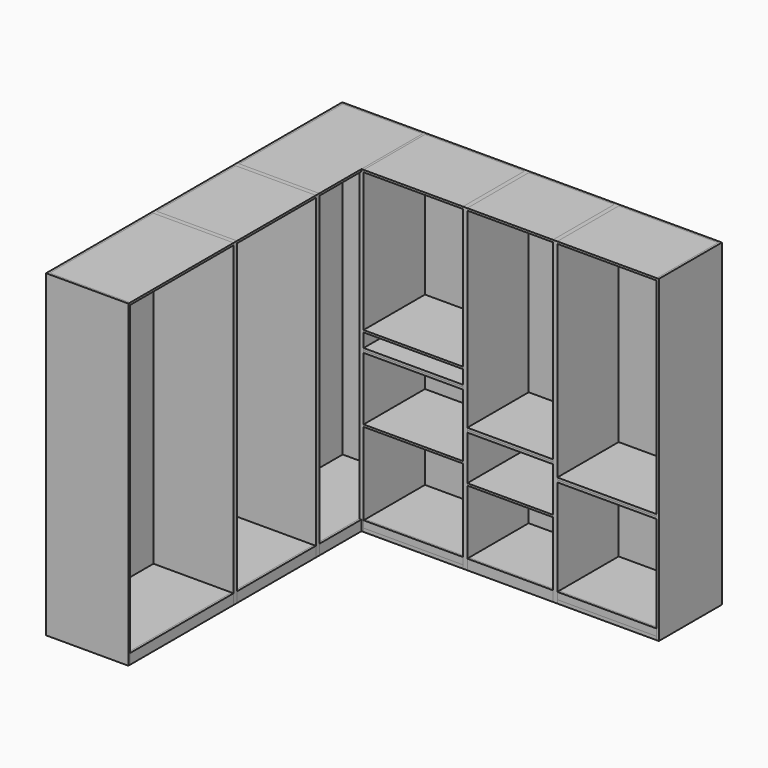
from build123d import *

# Parameters (mm, degrees)
F0_W      = 577.85
F0_H      = 730.25
F1_DEPTH  = 15.875
F0_W_2    = 736.6
F0_H_2    = 552.45
F0_W_3    = 635
F0_W_4    = 15.875
F0_H_3    = 958.85
F0_H_4    = 568.325
F0_H_5    = 15.875
F2_DEPTH  = 2362.2
F0_H_6    = 390.525
F3_DEPTH  = 76.2
F4_START  = 60.325
F4_DEPTH  = 15.875
F5_START  = 2346.325
F5_DEPTH  = 15.875
F6_DEPTH  = 25.4
F7_START  = 685.8
F7_DEPTH  = 15.875
F8_START  = 1168.4
F8_DEPTH  = 15.875
F9_START  = 1184.275
F9_DEPTH  = 15.875
F10_START = 1301.75
F10_DEPTH = 15.875
F11_START = 552.45
F11_DEPTH = 15.875
F12_START = 898.525
F12_DEPTH = 15.875
F13_START = 914.4
F13_DEPTH = 15.875
F14_DEPTH = 25.4
F15_START = 790.575
F15_DEPTH = 15.875
F16_START = 806.45
F16_DEPTH = 15.875
F17_R     = 12.7
F18_DEPTH = 768.35


# Not quite as in the source:
# - the program builds the solid bodies; features that only make, move or delete a surface that nothing else refers to are left out


with BuildPart() as f1:
    # F0 (on Top) → F1 (new body)
    with BuildSketch(Plane.XY):
        with Locations((-688.975, -1079.5)):
            Rectangle(F0_W, F0_H)
    extrude(amount=F1_DEPTH)


with BuildPart() as f1b:
    # F0 (on Top) → F1, piece 2 (new body)
    with BuildSketch(Plane.XY):
        Polygon((-400.05, -1866.9), (-400.05, -1476.375), (-977.9, -1476.375), (-977.9, -2435.225), (-400.05, -2435.225), align=None)
    extrude(amount=F1_DEPTH)


with BuildPart() as f1c:
    # F0 (on Top) → F1, piece 3 (new body)
    with BuildSketch(Plane.XY):
        Polygon((-400.05, -292.1), (-400.05, 276.225), (-977.9, 276.225), (-977.9, -682.625), (-400.05, -682.625), align=None)
    extrude(amount=F1_DEPTH)


with BuildPart() as f1d:
    # F0 (on Top) → F1, piece 4 (new body)
    with BuildSketch(Plane.XY):
        Rectangle(F0_W_2, F0_H_2)
    extrude(amount=F1_DEPTH)


with BuildPart() as f1e:
    # F0 (on Top) → F1, piece 5 (new body)
    with BuildSketch(Plane.XY):
        with Locations((717.55, 0)):
            Rectangle(F0_W_3, F0_H_2)
    extrude(amount=F1_DEPTH)


with BuildPart() as f1f:
    # F0 (on Top) → F1, piece 6 (new body)
    with BuildSketch(Plane.XY):
        with Locations((1435.1, 0)):
            Rectangle(F0_W_2, F0_H_2)
    extrude(amount=F1_DEPTH)


with BuildPart() as f2:
    # F0 (on Top) → F2 (new body)
    with BuildSketch(Plane.XY):
        Polygon((-977.9, -2435.225), (-993.775, -2435.225), (-993.775, -2451.1), (-384.175, -2451.1), (-384.175, -2435.225), (-400.05, -2435.225), align=None)
        with Locations((-985.8375, -1955.8)):
            Rectangle(F0_W_4, F0_H_3)
        Polygon((-384.175, -1476.375), (-384.175, -1460.5), (-993.775, -1460.5), (-993.775, -1476.375), (-977.9, -1476.375), (-400.05, -1476.375), align=None)
        Polygon((-384.175, -1460.5), (-384.175, -1444.625), (-400.05, -1444.625), (-977.9, -1444.625), (-993.775, -1444.625), (-993.775, -1460.5), align=None)
        with Locations((-985.8375, -1079.5)):
            Rectangle(F0_W_4, F0_H)
        Polygon((-384.175, -714.375), (-384.175, -698.5), (-993.775, -698.5), (-993.775, -714.375), (-977.9, -714.375), (-400.05, -714.375), align=None)
        Polygon((-384.175, -698.5), (-384.175, -682.625), (-400.05, -682.625), (-977.9, -682.625), (-993.775, -682.625), (-993.775, -698.5), align=None)
        with Locations((-392.1125, -7.9375)):
            Rectangle(F0_W_4, F0_H_4)
        Polygon((-368.3, 276.225), (-368.3, 292.1), (-384.175, 292.1), (-384.175, 276.225), (-384.175, -292.1), (-368.3, -292.1), (-368.3, -276.225), align=None)
        with Locations((-985.8375, -203.2)):
            Rectangle(F0_W_4, F0_H_3)
        Polygon((-384.175, 276.225), (-384.175, 292.1), (-993.775, 292.1), (-993.775, 276.225), (-977.9, 276.225), (-400.05, 276.225), align=None)
        with Locations((0, 284.1625)):
            Rectangle(F0_W_2, F0_H_5)
        Polygon((384.175, -292.1), (384.175, 292.1), (368.3, 292.1), (368.3, 276.225), (368.3, -276.225), (368.3, -292.1), align=None)
        Polygon((400.05, 292.1), (384.175, 292.1), (384.175, -292.1), (400.05, -292.1), (400.05, -276.225), (400.05, 276.225), align=None)
        with Locations((717.55, 284.1625)):
            Rectangle(F0_W_3, F0_H_5)
        Polygon((1050.925, 292.1), (1035.05, 292.1), (1035.05, 276.225), (1035.05, -276.225), (1035.05, -292.1), (1050.925, -292.1), align=None)
        Polygon((1066.8, 292.1), (1050.925, 292.1), (1050.925, -292.1), (1066.8, -292.1), (1066.8, -276.225), (1066.8, 276.225), align=None)
        with Locations((1435.1, 284.1625)):
            Rectangle(F0_W_2, F0_H_5)
        Polygon((1819.275, 292.1), (1803.4, 292.1), (1803.4, 276.225), (1803.4, -276.225), (1803.4, -292.1), (1819.275, -292.1), align=None)
    extrude(amount=F2_DEPTH)

    # F0 (on Top) → F15 (join)
    with BuildSketch(Plane.XY.offset(F15_START)):
        with Locations((1435.1, 0)):
            Rectangle(F0_W_2, F0_H_2)
        with Locations((1435.1, -284.1625)):
            Rectangle(F0_W_2, F0_H_5)
    extrude(amount=F15_DEPTH)

    # F17 (on face) → F18 (join)
    with BuildSketch(Plane.YZ.offset(1819.275)):
        with Locations((0, 2199.675321579)):
            Circle(F17_R)
    extrude(amount=-F18_DEPTH)


with BuildPart() as f3:
    # F0 (on Top) → F3 (new body)
    with BuildSketch(Plane.XY):
        with Locations((-392.1125, -2151.0625)):
            Rectangle(F0_W_4, F0_H_4)
        with Locations((-392.1125, -1671.6375)):
            Rectangle(F0_W_4, F0_H_6)
    extrude(amount=F3_DEPTH)


with BuildPart() as f3b:
    # F0 (on Top) → F3, piece 2 (new body)
    with BuildSketch(Plane.XY):
        with Locations((-392.1125, -1079.5)):
            Rectangle(F0_W_4, F0_H)
    extrude(amount=F3_DEPTH)


with BuildPart() as f3c:
    # F0 (on Top) → F3, piece 3 (new body)
    with BuildSketch(Plane.XY):
        with Locations((-392.1125, -487.3625)):
            Rectangle(F0_W_4, F0_H_6)
    extrude(amount=F3_DEPTH)


with BuildPart() as f3d:
    # F0 (on Top) → F3, piece 4 (new body)
    with BuildSketch(Plane.XY):
        with Locations((0, -284.1625)):
            Rectangle(F0_W_2, F0_H_5)
    extrude(amount=F3_DEPTH)


with BuildPart() as f3e:
    # F0 (on Top) → F3, piece 5 (new body)
    with BuildSketch(Plane.XY):
        with Locations((717.55, -284.1625)):
            Rectangle(F0_W_3, F0_H_5)
    extrude(amount=F3_DEPTH)


with BuildPart() as f3f:
    # F0 (on Top) → F3, piece 6 (new body)
    with BuildSketch(Plane.XY):
        with Locations((1435.1, -284.1625)):
            Rectangle(F0_W_2, F0_H_5)
    extrude(amount=F3_DEPTH)


with BuildPart() as f4:
    # F0 (on Top) → F4 (new body)
    with BuildSketch(Plane.XY.offset(F4_START)):
        Polygon((-400.05, -1866.9), (-400.05, -1476.375), (-977.9, -1476.375), (-977.9, -2435.225), (-400.05, -2435.225), align=None)
    extrude(amount=F4_DEPTH)


with BuildPart() as f4b:
    # F0 (on Top) → F4, piece 2 (new body)
    with BuildSketch(Plane.XY.offset(F4_START)):
        with Locations((-688.975, -1079.5)):
            Rectangle(F0_W, F0_H)
    extrude(amount=F4_DEPTH)


with BuildPart() as f4c:
    # F0 (on Top) → F4, piece 3 (new body)
    with BuildSketch(Plane.XY.offset(F4_START)):
        Polygon((-400.05, -292.1), (-400.05, 276.225), (-977.9, 276.225), (-977.9, -682.625), (-400.05, -682.625), align=None)
    extrude(amount=F4_DEPTH)


with BuildPart() as f4d:
    # F0 (on Top) → F4, piece 4 (new body)
    with BuildSketch(Plane.XY.offset(F4_START)):
        Rectangle(F0_W_2, F0_H_2)
    extrude(amount=F4_DEPTH)


with BuildPart() as f4e:
    # F0 (on Top) → F4, piece 5 (new body)
    with BuildSketch(Plane.XY.offset(F4_START)):
        with Locations((717.55, 0)):
            Rectangle(F0_W_3, F0_H_2)
    extrude(amount=F4_DEPTH)


with BuildPart() as f4f:
    # F0 (on Top) → F4, piece 6 (new body)
    with BuildSketch(Plane.XY.offset(F4_START)):
        with Locations((1435.1, 0)):
            Rectangle(F0_W_2, F0_H_2)
    extrude(amount=F4_DEPTH)


with BuildPart() as f5:
    # F0 (on Top) → F5 (new body)
    with BuildSketch(Plane.XY.offset(F5_START)):
        with Locations((-392.1125, -2151.0625)):
            Rectangle(F0_W_4, F0_H_4)
        with Locations((-392.1125, -1671.6375)):
            Rectangle(F0_W_4, F0_H_6)
        Polygon((-400.05, -1866.9), (-400.05, -1476.375), (-977.9, -1476.375), (-977.9, -2435.225), (-400.05, -2435.225), align=None)
    extrude(amount=F5_DEPTH)


with BuildPart() as f5b:
    # F0 (on Top) → F5, piece 2 (new body)
    with BuildSketch(Plane.XY.offset(F5_START)):
        with Locations((-392.1125, -1079.5)):
            Rectangle(F0_W_4, F0_H)
        with Locations((-688.975, -1079.5)):
            Rectangle(F0_W, F0_H)
    extrude(amount=F5_DEPTH)


with BuildPart() as f5c:
    # F0 (on Top) → F5, piece 3 (new body)
    with BuildSketch(Plane.XY.offset(F5_START)):
        with Locations((-392.1125, -7.9375)):
            Rectangle(F0_W_4, F0_H_4)
        with Locations((-392.1125, -487.3625)):
            Rectangle(F0_W_4, F0_H_6)
        Polygon((-400.05, -292.1), (-400.05, 276.225), (-977.9, 276.225), (-977.9, -682.625), (-400.05, -682.625), align=None)
    extrude(amount=F5_DEPTH)


with BuildPart() as f5d:
    # F0 (on Top) → F5, piece 4 (new body)
    with BuildSketch(Plane.XY.offset(F5_START)):
        with Locations((0, -284.1625)):
            Rectangle(F0_W_2, F0_H_5)
        Rectangle(F0_W_2, F0_H_2)
    extrude(amount=F5_DEPTH)


with BuildPart() as f5e:
    # F0 (on Top) → F5, piece 5 (new body)
    with BuildSketch(Plane.XY.offset(F5_START)):
        with Locations((717.55, -284.1625)):
            Rectangle(F0_W_3, F0_H_5)
        with Locations((717.55, 0)):
            Rectangle(F0_W_3, F0_H_2)
    extrude(amount=F5_DEPTH)


with BuildPart() as f5f:
    # F0 (on Top) → F5, piece 6 (new body)
    with BuildSketch(Plane.XY.offset(F5_START)):
        with Locations((1435.1, -284.1625)):
            Rectangle(F0_W_2, F0_H_5)
        with Locations((1435.1, 0)):
            Rectangle(F0_W_2, F0_H_2)
    extrude(amount=F5_DEPTH)


with BuildPart() as f6:
    # F0 (on Top) → F6 (new body)
    with BuildSketch(Plane.XY):
        with Locations((0, -284.1625)):
            Rectangle(F0_W_2, F0_H_5)
        Rectangle(F0_W_2, F0_H_2)
    extrude(amount=F6_DEPTH)


with BuildPart() as f7:
    # F0 (on Top) → F7 (new body)
    with BuildSketch(Plane.XY.offset(F7_START)):
        Rectangle(F0_W_2, F0_H_2)
        with Locations((0, -284.1625)):
            Rectangle(F0_W_2, F0_H_5)
    extrude(amount=F7_DEPTH)


with BuildPart() as f8:
    # F0 (on Top) → F8 (new body)
    with BuildSketch(Plane.XY.offset(F8_START)):
        with Locations((0, -284.1625)):
            Rectangle(F0_W_2, F0_H_5)
        Rectangle(F0_W_2, F0_H_2)
    extrude(amount=F8_DEPTH)


with BuildPart() as f9:
    # F0 (on Top) → F9 (new body)
    with BuildSketch(Plane.XY.offset(F9_START)):
        with Locations((0, -284.1625)):
            Rectangle(F0_W_2, F0_H_5)
        Rectangle(F0_W_2, F0_H_2)
    extrude(amount=F9_DEPTH)


with BuildPart() as f10:
    # F0 (on Top) → F10 (new body)
    with BuildSketch(Plane.XY.offset(F10_START)):
        Rectangle(F0_W_2, F0_H_2)
        with Locations((0, -284.1625)):
            Rectangle(F0_W_2, F0_H_5)
    extrude(amount=F10_DEPTH)


with BuildPart() as f11:
    # F0 (on Top) → F11 (new body)
    with BuildSketch(Plane.XY.offset(F11_START)):
        with Locations((717.55, -284.1625)):
            Rectangle(F0_W_3, F0_H_5)
        with Locations((717.55, 0)):
            Rectangle(F0_W_3, F0_H_2)
    extrude(amount=F11_DEPTH)


with BuildPart() as f12:
    # F0 (on Top) → F12 (new body)
    with BuildSketch(Plane.XY.offset(F12_START)):
        with Locations((717.55, -284.1625)):
            Rectangle(F0_W_3, F0_H_5)
        with Locations((717.55, 0)):
            Rectangle(F0_W_3, F0_H_2)
    extrude(amount=F12_DEPTH)


with BuildPart() as f13:
    # F0 (on Top) → F13 (new body)
    with BuildSketch(Plane.XY.offset(F13_START)):
        with Locations((717.55, -284.1625)):
            Rectangle(F0_W_3, F0_H_5)
        with Locations((717.55, 0)):
            Rectangle(F0_W_3, F0_H_2)
    extrude(amount=F13_DEPTH)


with BuildPart() as f14:
    # F0 (on Top) → F14 (new body)
    with BuildSketch(Plane.XY):
        with Locations((1435.1, -284.1625)):
            Rectangle(F0_W_2, F0_H_5)
        with Locations((1435.1, 0)):
            Rectangle(F0_W_2, F0_H_2)
    extrude(amount=F14_DEPTH)


with BuildPart() as f16:
    # F0 (on Top) → F16 (new body)
    with BuildSketch(Plane.XY.offset(F16_START)):
        with Locations((1435.1, -284.1625)):
            Rectangle(F0_W_2, F0_H_5)
        with Locations((1435.1, 0)):
            Rectangle(F0_W_2, F0_H_2)
    extrude(amount=F16_DEPTH)


solid = Compound([f1.part, f1b.part, f1c.part, f1d.part, f1e.part, f1f.part, f2.part, f3.part, f3b.part, f3c.part, f3d.part, f3e.part, f3f.part, f4.part, f4b.part, f4c.part, f4d.part, f4e.part, f4f.part, f5.part, f5b.part, f5c.part, f5d.part, f5e.part, f5f.part, f6.part, f7.part, f8.part, f9.part, f10.part, f11.part, f12.part, f13.part, f14.part, f16.part])
